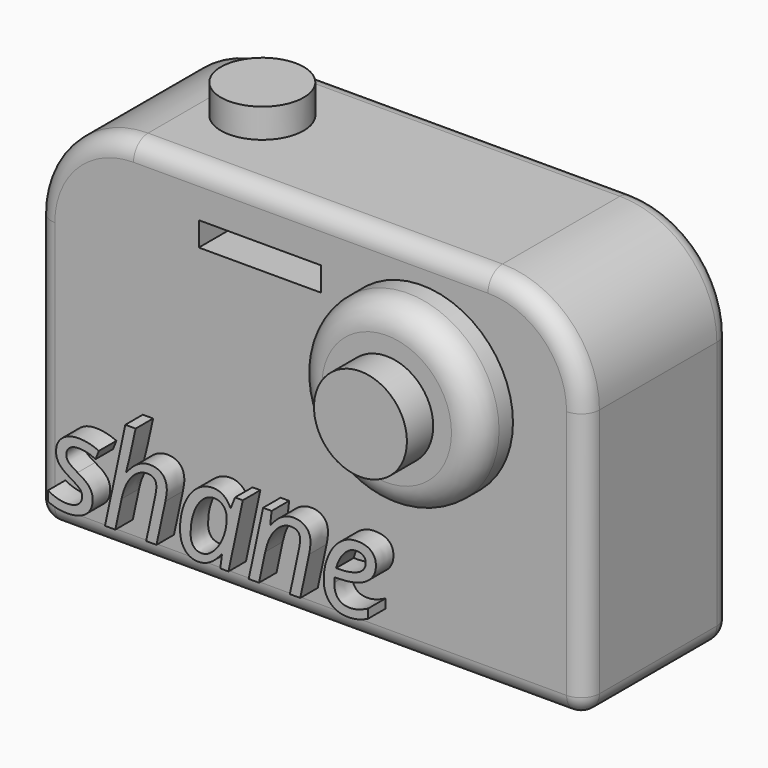
from build123d import *

# Parameters (mm, degrees)
F0_W         = 150.2221599221
F0_H         = 50.1984599978
F1_DEPTH     = 100
F2_R         = 26.5563491861
F3_R         = 5
F4_R         = 24.9868079134
F5_DEPTH     = 12
F6_R         = 11.3465245764
F7_DEPTH     = 8
F8_R         = 7.2426406871
F9_TEXT_SIZE = 34.466087042
F10_DEPTH    = 6
F11_W        = 33.466886729
F11_H        = 6.6023096442
F12_DEPTH    = 51
F13_W        = 104.7263070941
F13_H        = 57.8271346167
F14_DEPTH    = 9
F15_R        = 12.7322733561
F16_DEPTH    = 9


# Not quite as in the source:
# - Text() gives the source's letters only with a copy of the font that has no kerning and outlines rounded to 1/6400 em; it was checked with that copy


with BuildPart() as f1:
    # F0 (on Top) → F1 (new body)
    with BuildSketch(Plane.XY):
        with Locations((5.8782584965, 2.1460307762)):
            Rectangle(F0_W, F0_H)
    extrude(amount=F1_DEPTH)

    # F2
    f2_edges = [f1.edges().sort_by_distance(p)[0] for p in [
        (80.989338, 2.146031, 100),
        (-69.232821, 2.146031, 100),
    ]]
    fillet(f2_edges, radius=F2_R)

    # F3
    f3_edges = [f1.edges().sort_by_distance(p)[0] for p in [
        (-69.232821, 2.146031, 0),
        (80.989338, 2.146031, 0),
        (5.878258, -22.953199, 0),
        (5.878258, 27.245261, 0),
        (-69.232821, -22.953199, 36.721825),
        (-69.232821, 27.245261, 36.721825),
    ]]
    fillet(f3_edges, radius=F3_R)

    # F4 (on face) → F5 (join)
    with BuildSketch(Plane.XZ.offset(22.9531992227)):
        with Locations((36.3047979772, 66.0574659705)):
            Circle(F4_R)
    extrude(amount=F5_DEPTH)

    # F6 (on face) → F7 (join)
    with BuildSketch(Plane.XY.offset(100)):
        with Locations((-28.7292674184, 3.7322277203)):
            Circle(F6_R)
    extrude(amount=F7_DEPTH)

    # F8
    f8_edges = [f1.edges().sort_by_distance(p)[0] for p in [
        (11.31799, -34.953199, 66.057466),
    ]]
    fillet(f8_edges, radius=F8_R)

    # F9 (on face) → F10 (join)
    with BuildSketch(Plane.XZ.offset(22.9531992227)):
        with Locations((-61.4347755909, 8.7593598291)):
            Text('shane', F9_TEXT_SIZE, font='Open Sans', font_style=FontStyle.ITALIC, text_align=(TextAlign.LEFT, TextAlign.BOTTOM))
    extrude(amount=F10_DEPTH)

    # F11 (on face) → F12 (cut)
    with BuildSketch(Plane(origin=(0, 27.2452607751, 0), x_dir=(-1, 0, 0), z_dir=(0, 1, 0))):
        with Locations((8.0471280962, 83.547603339)):
            Rectangle(F11_W, F11_H)
    extrude(amount=-F12_DEPTH, mode=Mode.SUBTRACT)

    # F13 (on face) → F14 (cut)
    with BuildSketch(Plane(origin=(0, 27.2452607751, 0), x_dir=(-1, 0, 0), z_dir=(0, 1, 0))):
        with Locations((-2.9946677387, 38.8112566434)):
            Rectangle(F13_W, F13_H)
    extrude(amount=-F14_DEPTH, mode=Mode.SUBTRACT)

    # F15 (on face) → F16 (join)
    with BuildSketch(Plane.XZ.offset(34.9531992227)):
        with Locations((36.3047979772, 66.0574659705)):
            Circle(F15_R)
    extrude(amount=F16_DEPTH)


solid = f1.part
